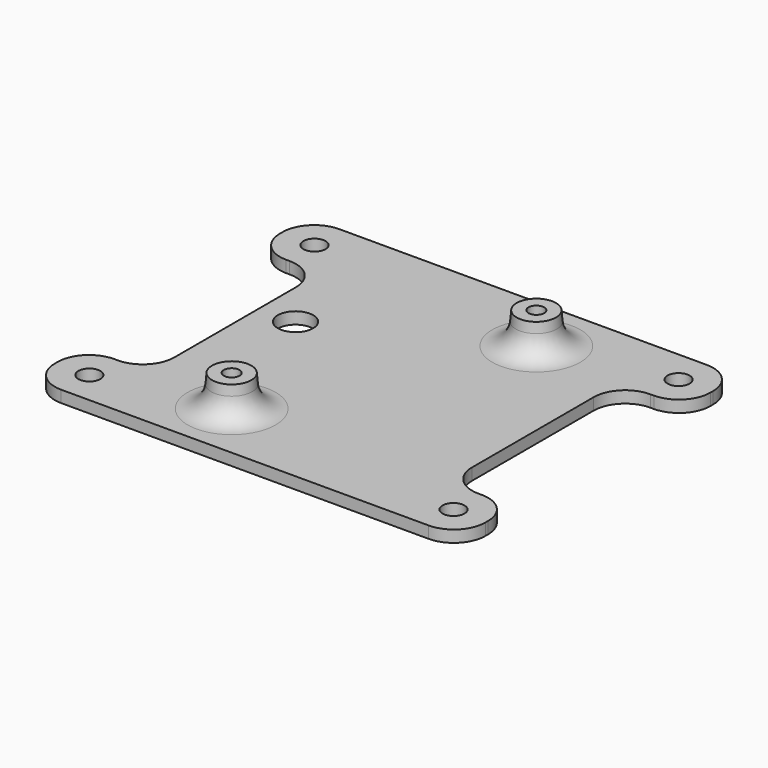
from build123d import *

# Parameters (mm, degrees)
F1_W     = 54.708
F1_H     = 77.4
F2_DEPTH = 1.5
F3_W     = 8.434
F3_H     = 27.322
F3_R     = 1.4
F3_R_2   = 1
F3_R_3   = 2.25
F4_DEPTH = 1.501
F5_R     = 4
F6_R     = 3
F6_R_2   = 1
F7_DEPTH = 4
F9_R     = 3


# Not quite as in the source:
# - a fillet or chamfer that OpenCascade refuses, or shapes differently, is made with other operations: its cross-section is extruded or revolved along the edge and cut away or added


with BuildPart() as f2:
    # F1 (on face) → F2 (new body)
    with BuildSketch(Plane.XY):
        with Locations((25.654, 37)):
            Rectangle(F1_W, F1_H)
    extrude(amount=F2_DEPTH)

    # F3 (on face) → F4 (cut, through all)
    with BuildSketch(Plane.XY.offset(1.5)):
        Polygon((44.574, 16.81), (6.734, 16.81), (-1.7, 16.81), (-1.7, -1.7), (53.008, -1.7), (53.008, 16.81), align=None)
        with Locations((2.517, 38.905)):
            Rectangle(F3_W, F3_H)
        with Locations((48.791, 38.905)):
            Rectangle(F3_W, F3_H)
        Polygon((-1.7, 61), (6.734, 61), (44.574, 61), (53.008, 61), (53.008, 75.7), (-1.7, 75.7), align=None)
        with Locations((2.517, 21.027)):
            Circle(F3_R)
        with Locations((48.791, 21.027)):
            Circle(F3_R)
        with Locations((48.791, 56.783)):
            Circle(F3_R)
        with Locations((2.517, 56.783)):
            Circle(F3_R)
        with Locations((33.254, 53.605)):
            Circle(F3_R_2)
        with Locations((18.054, 24.205)):
            Circle(F3_R_2)
        with Locations((11.334, 42.75)):
            Circle(F3_R_3)
    extrude(amount=-F4_DEPTH, mode=Mode.SUBTRACT)

    # F5
    f5_edges = [f2.edges().sort_by_distance(p)[0] for p in [
        (-1.7, 61, 0.75),
        (-1.7, 52.566, 0.75),
        (-1.7, 25.244, 0.75),
        (-1.7, 16.81, 0.75),
        (6.734, 25.244, 0.75),
        (6.734, 52.566, 0.75),
        (53.008, 61, 0.75),
        (53.008, 52.566, 0.75),
        (44.574, 52.566, 0.75),
        (44.574, 25.244, 0.75),
        (53.008, 25.244, 0.75),
        (53.008, 16.81, 0.75),
    ]]
    fillet(f5_edges, radius=F5_R)

    # F6 (on face) → F7 (join)
    with BuildSketch(Plane.XY.offset(1.5)):
        with Locations((18.054, 24.205)):
            Circle(F6_R)
        with Locations((18.054, 24.205)):
            Circle(F6_R_2, mode=Mode.SUBTRACT)
        with Locations((33.254, 53.605)):
            Circle(F6_R)
        with Locations((33.254, 53.605)):
            Circle(F6_R_2, mode=Mode.SUBTRACT)
    extrude(amount=F7_DEPTH)

    # F8: chamfer of 0.5 x 5.7150261514 on 2 edges, made by hand


with BuildPart() as f8_tool2:
    # F8_s3 → F8_t4 (revolve)
    with BuildSketch(Plane.XZ.offset(-24.205)):
        Polygon((21.054, -0.2150261514), (20.554, 5.5), (21.054, 5.5), align=None)
    revolve(axis=Axis((18.054, 24.205, 5.5), (0, 0, 1)))

    split(bisect_by=Plane.XY.offset(1.5), keep=Keep.TOP)


with BuildPart() as f2_1:
    add(f2.part)

    # F8_t1: cut F8_tool2
    add(f8_tool2.part, mode=Mode.SUBTRACT)


with BuildPart() as f8_tool7:
    # F8_s8 → F8_t9 (revolve)
    with BuildSketch(Plane.XZ.offset(-53.605)):
        Polygon((36.254, -0.2150261514), (35.754, 5.5), (36.254, 5.5), align=None)
    revolve(axis=Axis((33.254, 53.605, 5.5), (0, 0, 1)))

    split(bisect_by=Plane.XY.offset(1.5), keep=Keep.TOP)


with BuildPart() as f2_2:
    add(f2_1.part)

    # F8_t6: cut F8_tool7
    add(f8_tool7.part, mode=Mode.SUBTRACT)

    # F9
    f9_edges = [f2_2.edges().sort_by_distance(p)[0] for p in [
        (15.204045, 24.205, 1.5),
        (30.404045, 53.605, 1.5),
    ]]
    fillet(f9_edges, radius=F9_R)


solid = f2_2.part
